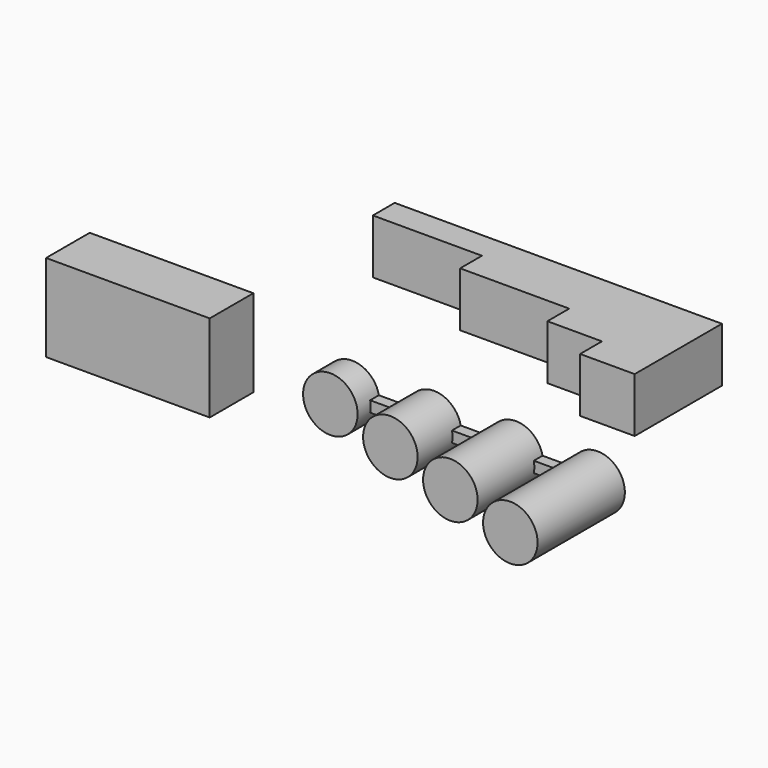
from build123d import *

# Parameters (mm, degrees)
F0_R      = 5
F1_DEPTH  = 5
F2_DEPTH  = 10
F3_DEPTH  = 15
F4_DEPTH  = 20
F7_W      = 60
F7_H      = 10
F8_DEPTH  = 5
F9_W      = 40
F9_H      = 10
F10_DEPTH = 5
F11_W     = 20
F11_H     = 10
F12_DEPTH = 5
F13_W     = 10
F13_H     = 10
F14_DEPTH = 5
F15_W     = 44.9199787766
F15_H     = 2
F16_DEPTH = 2
F17_W     = 30
F17_H     = 10
F18_DEPTH = 16


# Not quite as in the source:
# - a feature names something its author has since deleted; it is built from what else it names


with BuildPart() as f1:
    # F0 (on Front) → F1 (new body)
    with BuildSketch(Plane.XZ):
        Circle(F0_R)
    extrude(amount=F1_DEPTH)


with BuildPart() as f2:
    # F0 (on Front) → F2 (new body)
    with BuildSketch(Plane.XZ):
        with Locations((15, 0)):
            Circle(F0_R)
    extrude(amount=F2_DEPTH)


with BuildPart() as f3:
    # F0 (on Front) → F3 (new body)
    with BuildSketch(Plane.XZ):
        with Locations((30, 0)):
            Circle(F0_R)
    extrude(amount=F3_DEPTH)


with BuildPart() as f4:
    # F0 (on Front) → F4 (new body)
    with BuildSketch(Plane.XZ):
        with Locations((45, 0)):
            Circle(F0_R)
    extrude(amount=F4_DEPTH)

    # F6: union F3, F2, F1
    add(f3.part)
    add(f2.part)
    add(f1.part)

    # F15 (on face) → F16 (join)
    with BuildSketch(Plane.XZ):
        with Locations((22.7489862844, 0)):
            Rectangle(F15_W, F15_H)
    extrude(amount=F16_DEPTH)


with BuildPart() as f8:
    # F7 (on face) → F8 (new body)
    with BuildSketch(Plane(origin=(0, 0, 0), x_dir=(-1, 0, 0), z_dir=(0, 1, 0))):
        with Locations((-37.7946806746, 27.9940228151)):
            Rectangle(F7_W, F7_H)
    extrude(amount=-F8_DEPTH)

    # F9 (on face) → F10 (join)
    with BuildSketch(Plane.XZ.offset(5)):
        with Locations((47.7946806746, 27.9940228151)):
            Rectangle(F9_W, F9_H)
    extrude(amount=F10_DEPTH)

    # F11 (on face) → F12 (join)
    with BuildSketch(Plane.XZ.offset(10)):
        with Locations((57.7946806746, 27.9940228151)):
            Rectangle(F11_W, F11_H)
    extrude(amount=F12_DEPTH)

    # F13 (on face) → F14 (join)
    with BuildSketch(Plane.XZ.offset(15)):
        with Locations((62.7946806746, 27.9940228151)):
            Rectangle(F13_W, F13_H)
    extrude(amount=F14_DEPTH)


with BuildPart() as f18:
    # F17 (on Top) → F18 (new body)
    with BuildSketch(Plane.XY):
        with Locations((-25.8990339628, -14.026532881)):
            Rectangle(F17_W, F17_H)
    extrude(amount=F18_DEPTH)


solid = Compound([f4.part, f8.part, f18.part])
